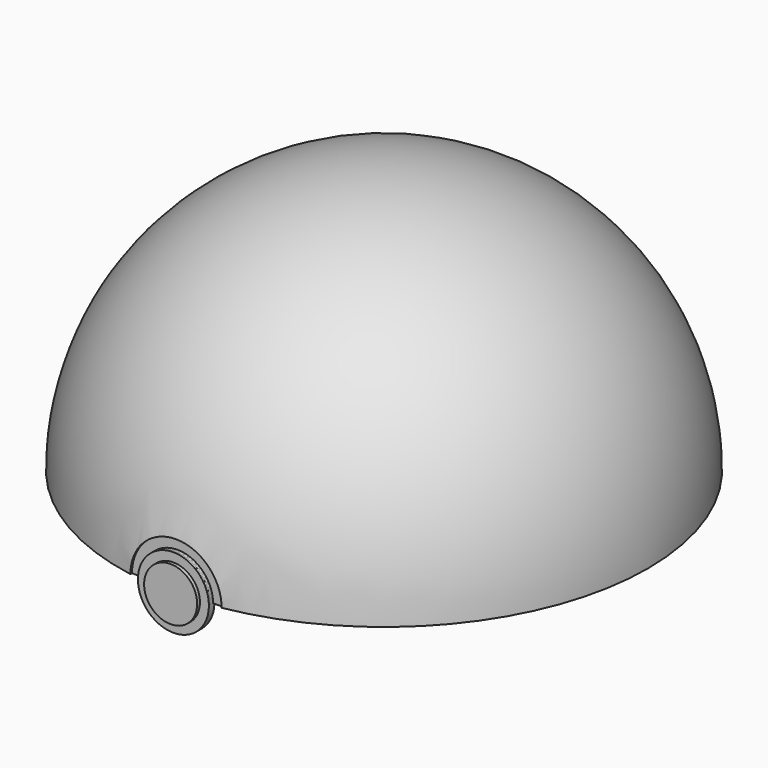
from build123d import *

# Parameters (mm, degrees)
F1_ANGLE_BACK = 90
F1_ANGLE      = 180
F2_T          = -2.5
F3_R          = 10.2502002621
F4_DEPTH      = 74
F5_R          = 10.2502002621
F6_DEPTH      = 2
F7_R          = 7.6569283782
F8_DEPTH      = 1
F9_R          = 13.1650380961
F9_R_2        = 10.2502002621
F10_DEPTH     = 1.5


# Not quite as in the source:
# - ends of sketch curves that miss each other by under 0.0002 mm in the source are joined


with BuildPart() as f1:
    # F0 (on Front) → F1 (revolve)
    with BuildSketch(Plane.XZ, mode=Mode.PRIVATE) as f1_sk:
        with BuildLine():
            ThreePointArc((76.1996501387, 4.35119e-05), (3.66272e-05, 76.1996570235), (-76.1995768844, 4.35119e-05))
            Line((-76.1995768844, 4.35119e-05), (76.1996501387, 4.35119e-05))
        make_face()
    revolve(f1_sk.sketch.rotate(Axis((8.50559e-05, 0, 4.35119e-05), (-1, 0, 0)), -F1_ANGLE_BACK), axis=Axis((8.50559e-05, 0, 4.35119e-05), (-1, 0, 0)), revolution_arc=F1_ANGLE)

    # F2
    f2_openings = [f1.faces().sort_by_distance(p)[0] for p in [
        (3.7e-05, 0, 4.4e-05),
    ]]
    offset(amount=F2_T, openings=f2_openings)

    # F9 (on face) → F10 (cut)
    with BuildSketch(Plane.XZ.offset(76)):
        Circle(F9_R)
        Circle(F9_R_2, mode=Mode.SUBTRACT)
    extrude(amount=-F10_DEPTH, mode=Mode.SUBTRACT)


with BuildPart() as f4:
    # F3 (on Front) → F4 (new body)
    with BuildSketch(Plane.XZ):
        Circle(F3_R)
    extrude(amount=F4_DEPTH)


with BuildPart() as f6:
    # F5 (on face) → F6 (new body)
    with BuildSketch(Plane.XZ.offset(74)):
        Circle(F5_R)
    extrude(amount=F6_DEPTH)

    # F7 (on face) → F8 (join)
    with BuildSketch(Plane.XZ.offset(76)):
        Circle(F7_R)
    extrude(amount=F8_DEPTH)


solid = Compound([f1.part, f6.part])
